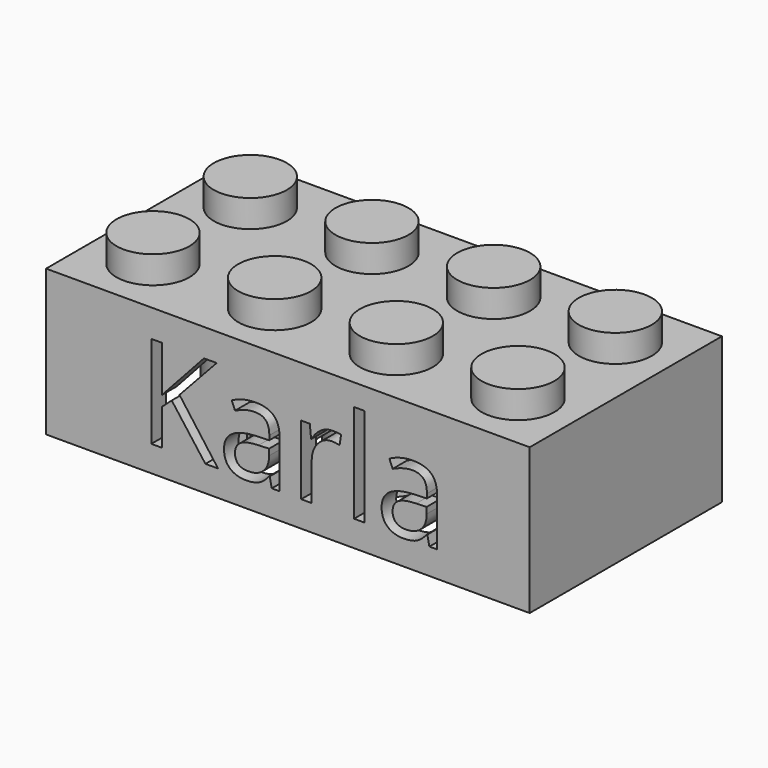
from build123d import *

# Parameters (mm, degrees)
F0_W          = 31.8
F0_H          = 15.8
F1_DEPTH      = 9.6
F2_W          = 29.4
F2_H          = 13.4
F3_DEPTH      = 8.4
F4_R          = 2.4
F5_DEPTH      = 1.8
F6_R          = 1.3
F7_DEPTH      = 1.2
F8_R          = 3.255
F8_R_2        = 2.4
F9_DEPTH      = 8.4
F10_W         = 0.6
F10_H         = 0.3
F11_DEPTH     = 8.4
F12_W         = 0.3
F12_H         = 0.6
F13_DEPTH     = 8.4
F14_W         = 0.6
F14_H         = 4.25
F14_H_2       = 4.2500009078
F15_DEPTH     = 4.2
F16_TEXT_SIZE = 8.5133483582
F17_DEPTH     = 1.2


# Not quite as in the source:
# - Text() gives the source's letters only with a copy of the font that has no kerning and outlines rounded to 1/6400 em; it was checked with that copy


with BuildPart() as f1:
    # F0 (on Top) → F1 (new body)
    with BuildSketch(Plane.XY):
        Rectangle(F0_W, F0_H)
    extrude(amount=F1_DEPTH)

    # F2 (on face) → F3 (cut)
    with BuildSketch(Plane(origin=(0, 0, 0), x_dir=(1, 0, 0), z_dir=(0, 0, -1))):
        Rectangle(F2_W, F2_H)
    extrude(amount=-F3_DEPTH, mode=Mode.SUBTRACT)

    # F4 (on face) → F5 (join)
    with BuildSketch(Plane.XY.offset(9.6)):
        with Locations((-11.95, 3.95)):
            Circle(F4_R)
        with Locations((-11.95, -4.05)):
            Circle(F4_R)
        with Locations((-3.95, 3.95)):
            Circle(F4_R)
        with Locations((-3.95, -4.05)):
            Circle(F4_R)
        with Locations((4.05, 3.95)):
            Circle(F4_R)
        with Locations((4.05, -4.05)):
            Circle(F4_R)
        with Locations((12.05, 3.95)):
            Circle(F4_R)
        with Locations((12.05, -4.05)):
            Circle(F4_R)
    extrude(amount=F5_DEPTH)

    # F6 (on face) → F7 (cut)
    with BuildSketch(Plane(origin=(0, 0, 8.4), x_dir=(1, 0, 0), z_dir=(0, 0, -1))):
        with Locations((-11.95, 3.95)):
            Circle(F6_R)
        with Locations((-11.95, -4.05)):
            Circle(F6_R)
        with Locations((-3.95, 3.95)):
            Circle(F6_R)
        with Locations((-3.95, -4.05)):
            Circle(F6_R)
        with Locations((4.05, 3.95)):
            Circle(F6_R)
        with Locations((4.05, -4.05)):
            Circle(F6_R)
        with Locations((12.05, 3.95)):
            Circle(F6_R)
        with Locations((12.05, -4.05)):
            Circle(F6_R)
    extrude(amount=-F7_DEPTH, mode=Mode.SUBTRACT)

    # F8 (on face) → F9 (join, through all)
    with BuildSketch(Plane(origin=(0, 0, 8.4), x_dir=(1, 0, 0), z_dir=(0, 0, -1))):
        with Locations((-7.95, -0.05)):
            Circle(F8_R)
        with Locations((-7.95, -0.05)):
            Circle(F8_R_2, mode=Mode.SUBTRACT)
        with Locations((0.05, -0.05)):
            Circle(F8_R)
        with Locations((0.05, -0.05)):
            Circle(F8_R_2, mode=Mode.SUBTRACT)
        with Locations((8.05, -0.05)):
            Circle(F8_R)
        with Locations((8.05, -0.05)):
            Circle(F8_R_2, mode=Mode.SUBTRACT)
    extrude(amount=F9_DEPTH)

    # F10 (on face) → F11 (join, through all)
    with BuildSketch(Plane(origin=(0, 0, 0), x_dir=(1, 0, 0), z_dir=(0, 0, -1))):
        with Locations((-11.95, 6.55)):
            Rectangle(F10_W, F10_H)
        with Locations((-11.95, -6.55)):
            Rectangle(F10_W, F10_H)
        with Locations((-3.95, 6.55)):
            Rectangle(F10_W, F10_H)
        with Locations((-3.95, -6.55)):
            Rectangle(F10_W, F10_H)
        with Locations((4.05, 6.55)):
            Rectangle(F10_W, F10_H)
        with Locations((4.05, -6.55)):
            Rectangle(F10_W, F10_H)
        with Locations((12.05, 6.55)):
            Rectangle(F10_W, F10_H)
        with Locations((12.05, -6.55)):
            Rectangle(F10_W, F10_H)
    extrude(amount=-F11_DEPTH)

    # F12 (on face) → F13 (join, through all)
    with BuildSketch(Plane(origin=(0, 0, 0), x_dir=(1, 0, 0), z_dir=(0, 0, -1))):
        with Locations((-14.55, 3.95)):
            Rectangle(F12_W, F12_H)
        with Locations((-14.55, -4.05)):
            Rectangle(F12_W, F12_H)
        with Locations((14.55, 3.95)):
            Rectangle(F12_W, F12_H)
        with Locations((14.55, -4.05)):
            Rectangle(F12_W, F12_H)
    extrude(amount=-F13_DEPTH)

    # F14 (on face) → F15 (join)
    with BuildSketch(Plane(origin=(0, 0, 8.4), x_dir=(1, 0, 0), z_dir=(0, 0, -1))):
        with Locations((0, 4.825)):
            Rectangle(F14_W, F14_H)
        with Locations((0, -4.8249995461)):
            Rectangle(F14_W, F14_H_2)
    extrude(amount=F15_DEPTH)

    # F16 (on face) → F17 (cut)
    with BuildSketch(Plane.XZ.offset(7.9)):
        with Locations((-9.8169548255, 1.7051887698)):
            Text('Karla', F16_TEXT_SIZE, font='Open Sans', text_align=(TextAlign.LEFT, TextAlign.BOTTOM))
    extrude(amount=-F17_DEPTH, mode=Mode.SUBTRACT)


solid = f1.part
